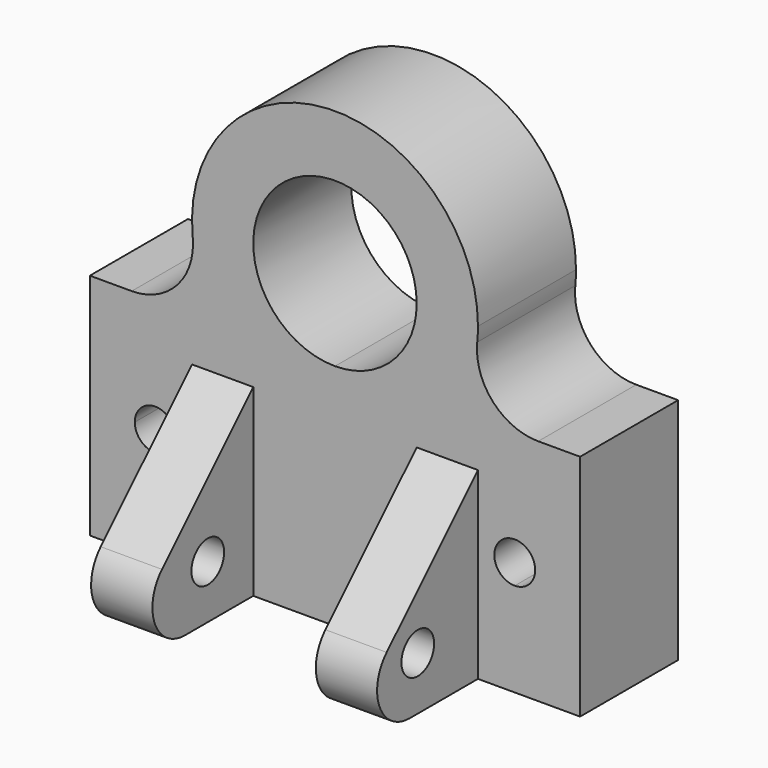
from build123d import *

# Parameters (mm, degrees)
F1_DEPTH = 30
F3_R     = 5
F4_DEPTH = 15
F5_R     = 10
F7_R     = 5
F8_DEPTH = 15
F9_R     = 10


# Not quite as in the source:
# - a feature names something its author has since deleted; it is built from what else it names


with BuildPart() as f1:
    # F0 (on Front) → F1 (new body)
    with BuildSketch(Plane.XZ):
        with BuildLine():
            Line((60, 0), (60, 28))
            Line((60, 28), (49.7493718553, 28))
            Line((49.7493718553, 28), (28.7228132327, 28))
            ThreePointArc((28.7228132327, 28), (0, 13), (-28.7228132327, 28))
            Line((-28.7228132327, 28), (-49.7493718553, 28))
            Line((-49.7493718553, 28), (-60, 28))
            Line((-60, 28), (-60, 0))
            Line((-60, 0), (-49, 0))
            ThreePointArc((-49, 0), (-44, 5), (-39, 0))
            ThreePointArc((-39, 0), (-40.4644660941, -3.5355339059), (-44, -5))
            Line((-44, -5), (-44, -28))
            Line((-44, -28), (44, -28))
            Line((44, -28), (44, -5))
            ThreePointArc((44, -5), (40.4644660941, 3.5355339059), (49, 0))
            Line((49, 0), (60, 0))
        make_face()
        with BuildLine():
            Line((-6.45e-08, 28), (28.7228132327, 28))
            ThreePointArc((28.7228132327, 28), (32.8272702395, 35.8603818585), (34.8245603048, 44.5000000607))
            ThreePointArc((34.8245603048, 44.5000000607), (34.9561125604, 46.2478029033), (35, 48))
            ThreePointArc((35, 48), (-1.7521970967, 82.9561125604), (-34.8245603048, 44.5000000607))
            ThreePointArc((-34.8245603048, 44.5000000607), (-32.8272702395, 35.8603818585), (-28.7228132327, 28))
            Line((-28.7228132327, 28), (-6.45e-08, 28))
        make_face()
        with BuildLine():
            ThreePointArc((20, 48), (14.1421356009, 33.8578643535), (-6.45e-08, 28))
            ThreePointArc((-6.45e-08, 28), (-14.1421356009, 62.1421356465), (20, 48))
        make_face(mode=Mode.SUBTRACT)
        with BuildLine():
            ThreePointArc((-28.7228132327, 28), (0, 13), (28.7228132327, 28))
            Line((28.7228132327, 28), (-6.45e-08, 28))
            Line((-6.45e-08, 28), (-28.7228132327, 28))
        make_face()
        with BuildLine():
            Line((-49.7493718553, 28), (-28.7228132327, 28))
            ThreePointArc((-28.7228132327, 28), (-32.8272702395, 35.8603818585), (-34.8245603048, 44.5000000607))
            ThreePointArc((-34.8245603048, 44.5000000607), (-34.7681807602, 43.7509416563), (-34.7493718553, 43))
            ThreePointArc((-34.7493718553, 43), (-39.1427701375, 32.3933982822), (-49.7493718553, 28))
        make_face()
        with BuildLine():
            Line((28.7228132327, 28), (49.7493718553, 28))
            ThreePointArc((49.7493718553, 28), (38.6250741042, 32.9376941239), (34.8245603048, 44.5000000607))
            ThreePointArc((34.8245603048, 44.5000000607), (32.8272702395, 35.8603818585), (28.7228132327, 28))
        make_face()
        with BuildLine():
            Line((-60, -28), (-44, -28))
            Line((-44, -28), (-44, -5))
            ThreePointArc((-44, -5), (-47.5355339059, -3.5355339059), (-49, 0))
            Line((-49, 0), (-60, 0))
            Line((-60, 0), (-60, -28))
        make_face()
        with BuildLine():
            Line((60, -28), (60, 0))
            Line((60, 0), (49, 0))
            ThreePointArc((49, 0), (47.5355339059, -3.5355339059), (44, -5))
            Line((44, -5), (44, -28))
            Line((44, -28), (60, -28))
        make_face()
    extrude(amount=F1_DEPTH)

    # F3 (on offset) → F4 (join)
    with BuildSketch(Plane.YZ.offset(20)):
        Polygon((-75, -28), (-30, -28), (-30, 17), align=None)
        with Locations((-48.4146624804, -14.9473380297)):
            Circle(F3_R, mode=Mode.SUBTRACT)
    extrude(amount=F4_DEPTH)

    # F5
    f5_edges = [f1.edges().sort_by_distance(p)[0] for p in [
        (27.5, -75, -28),
    ]]
    fillet(f5_edges, radius=F5_R)


with BuildPart() as f8:
    # F7 (on offset) → F8 (new body)
    with BuildSketch(Plane.YZ.offset(-20)):
        Polygon((-75, -28), (-30, -28), (-30, 17), align=None)
        with Locations((-43.9220774009, -14.9473380297)):
            Circle(F7_R, mode=Mode.SUBTRACT)
    extrude(amount=-F8_DEPTH)

    # F9
    f9_edges = [f8.edges().sort_by_distance(p)[0] for p in [
        (-27.5, -75, -28),
    ]]
    fillet(f9_edges, radius=F9_R)


solid = Compound([f1.part, f8.part])
